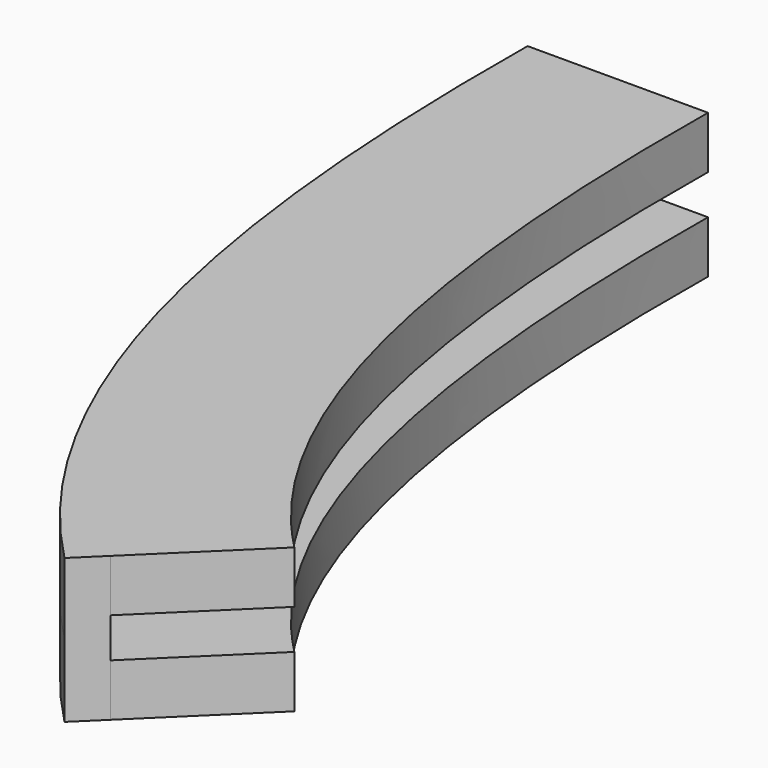
from build123d import *

# Parameters (mm, degrees)
F1_DEPTH = 10.16
F2_DEPTH = 2.794


# Not quite as in the source:
# - ends of sketch curves that miss each other by under 0.0002 mm in the source are joined


with BuildPart() as f1:
    # F0 (on Top) → F1 (new body, symmetric)
    with BuildSketch(Plane.XY):
        with BuildLine():
            add(Edge.make_bspline(
                [(-30.1686804344, 43.3476526069), (-30.8248162722, -8.7581067609), (-22.1361141771, -44.4161965277), (-1.0204318918, -65.8959671855)],
                knots=[14.1187831422, 14.1187831422, 14.1187831422, 14.1187831422, 131.8278556138, 131.8278556138, 131.8278556138, 131.8278556138], degree=3))
            Line((-30.1686804344, 43.3476526069), (-50.4902243697, 43.3476526069))
            add(Edge.make_bspline(
                [(-50.4902243697, 43.3476526069), (-50.5023356823, 42.3416381346), (-50.5776631638, 33.7575699347), (-50.2547042611, 18.2728647958), (-48.5490186564, -1.9094845449), (-45.4683930825, -20.5766183405), (-40.8513482733, -37.8029140743), (-34.4978508868, -53.6097599892), (-26.2151831057, -67.8904361601), (-19.3239866258, -76.2568786685), (-15.5576457112, -80.0936870299)],
                knots=[0.1084983974, 0.1084983974, 0.1084983974, 0.1084983974, 0.125, 0.25, 0.375, 0.5, 0.625, 0.75, 0.875, 0.9994876672, 0.9994876672, 0.9994876672, 0.9994876672], degree=3))
            Line((-15.5576457112, -80.0936870299), (-15.5504097194, -80.1010887171))
            Line((-15.5504097194, -80.1010887171), (-1.0204318918, -65.8959671855))
        make_face()
        with BuildLine():
            add(Edge.make_bspline(
                [(-50.4902243697, 43.3476526462), (-50.5023356823, 42.3416381346), (-50.5776631638, 33.7575699347), (-50.2547042611, 18.2728647958), (-48.5490186564, -1.9094845449), (-45.4683930825, -20.5766183405), (-40.8513482733, -37.8029140743), (-34.4978508868, -53.6097599892), (-26.2151831057, -67.8904361601), (-19.3239866258, -76.2568786685), (-15.5576457112, -80.0936870299)],
                knots=[0.1084983974, 0.1084983974, 0.1084983974, 0.1084983974, 0.125, 0.25, 0.375, 0.5, 0.625, 0.75, 0.875, 0.9994876672, 0.9994876672, 0.9994876672, 0.9994876672], degree=3))
            Line((-50.4902243697, 43.3476526462), (-55.5705854562, 43.3476526069))
            add(Edge.make_bspline(
                [(-55.5705854562, 43.3476526069), (-55.5824542112, 42.3512221988), (-55.6578660057, 33.6924970547), (-55.3319230242, 18.0236423903), (-53.5978680793, -2.5165326287), (-50.4470600065, -21.6261667001), (-45.6901847728, -39.3890823186), (-39.0903346211, -55.8222129569), (-30.4150960171, -70.7885790199), (-23.1570048132, -79.6038664954), (-19.1828818554, -83.6523472777)],
                knots=[0.1088294141, 0.1088294141, 0.1088294141, 0.1088294141, 0.125, 0.25, 0.375, 0.5, 0.625, 0.75, 0.875, 0.9994877133, 0.9994877133, 0.9994877133, 0.9994877133], degree=3))
            Line((-19.1828818554, -83.6523472777), (-15.5504097194, -80.1010887171))
            Line((-15.5504097194, -80.1010887171), (-15.5576457112, -80.0936870299))
        make_face()
    extrude(amount=F1_DEPTH, both=True)

    # F0 (on Top) → F2 (cut, symmetric)
    with BuildSketch(Plane.XY):
        with BuildLine():
            add(Edge.make_bspline(
                [(-30.1686804344, 43.3476526069), (-30.8248162722, -8.7581067609), (-22.1361141771, -44.4161965277), (-1.0204318918, -65.8959671855)],
                knots=[14.1187831422, 14.1187831422, 14.1187831422, 14.1187831422, 131.8278556138, 131.8278556138, 131.8278556138, 131.8278556138], degree=3))
            Line((-30.1686804344, 43.3476526069), (-50.4902243697, 43.3476526069))
            add(Edge.make_bspline(
                [(-50.4902243697, 43.3476526069), (-50.5023356823, 42.3416381346), (-50.5776631638, 33.7575699347), (-50.2547042611, 18.2728647958), (-48.5490186564, -1.9094845449), (-45.4683930825, -20.5766183405), (-40.8513482733, -37.8029140743), (-34.4978508868, -53.6097599892), (-26.2151831057, -67.8904361601), (-19.3239866258, -76.2568786685), (-15.5576457112, -80.0936870299)],
                knots=[0.1084983974, 0.1084983974, 0.1084983974, 0.1084983974, 0.125, 0.25, 0.375, 0.5, 0.625, 0.75, 0.875, 0.9994876672, 0.9994876672, 0.9994876672, 0.9994876672], degree=3))
            Line((-15.5576457112, -80.0936870299), (-15.5504097194, -80.1010887171))
            Line((-15.5504097194, -80.1010887171), (-1.0204318918, -65.8959671855))
        make_face()
    extrude(amount=F2_DEPTH, both=True, mode=Mode.SUBTRACT)


solid = f1.part
